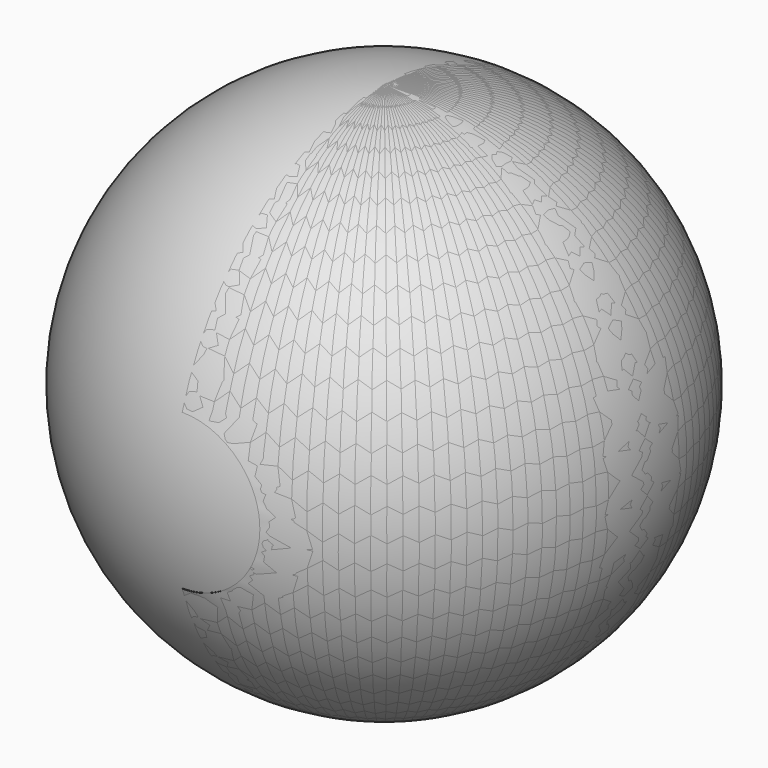
from build123d import *
from build123d import SkipClean  # not in build123d's __all__

# Parameters (mm, degrees)
F5_R          = 3.175
F6_DEPTH      = 10.796
F6_DEPTH_BACK = 10.796


with BuildPart() as f1:
    # F0 (on Front) → F1 (revolve)
    with BuildSketch(Plane.XZ):
        with BuildLine():
            Line((0, 10.795), (0, -10.795))
            ThreePointArc((0, -10.795), (10.795, 0), (0, 10.795))
        make_face()
    revolve(axis=Axis((0, 0, 0), (0, 0, -1)))


with BuildPart() as f2_1:
    # F2: copy of F1
    add(f1.part, clean=False)

    # F3 (on Front) → F4 (revolve, cut)
    with BuildSketch(Plane.XZ):
        with BuildLine():
            Line((0, 9.271), (0, 9.525))
            ThreePointArc((0, 9.525), (-6.7351920908, 6.7351920908), (-9.525, 0))
            Line((-9.525, 0), (0, 0))
            Line((0, 0), (0, 9.271))
        make_face()
        with BuildLine():
            ThreePointArc((-9.525, 0), (-6.7351920908, 6.7351920908), (0, 9.525))
            Line((0, 9.525), (0, 11.9412727654))
            ThreePointArc((0, 11.9412727654), (-8.6395970783, 8.6589956568), (-11.87035162, 0))
            Line((-11.87035162, 0), (-9.525, 0))
        make_face()
    with SkipClean():  # cleaning this boolean's faces spoils the solid; the shape is the same uncleaned
        revolve(axis=Axis((-4.7625, 0, 0), (-1, 0, 0)), mode=Mode.SUBTRACT)

    # F5 (on Front) → F6 (cut, two sides)
    with BuildSketch(Plane.XZ) as f6_sk:
        Circle(F5_R)
    extrude(amount=-F6_DEPTH, mode=Mode.SUBTRACT)
    extrude(f6_sk.sketch, amount=F6_DEPTH_BACK, mode=Mode.SUBTRACT)


solid = Compound([f1.part, f2_1.part])
